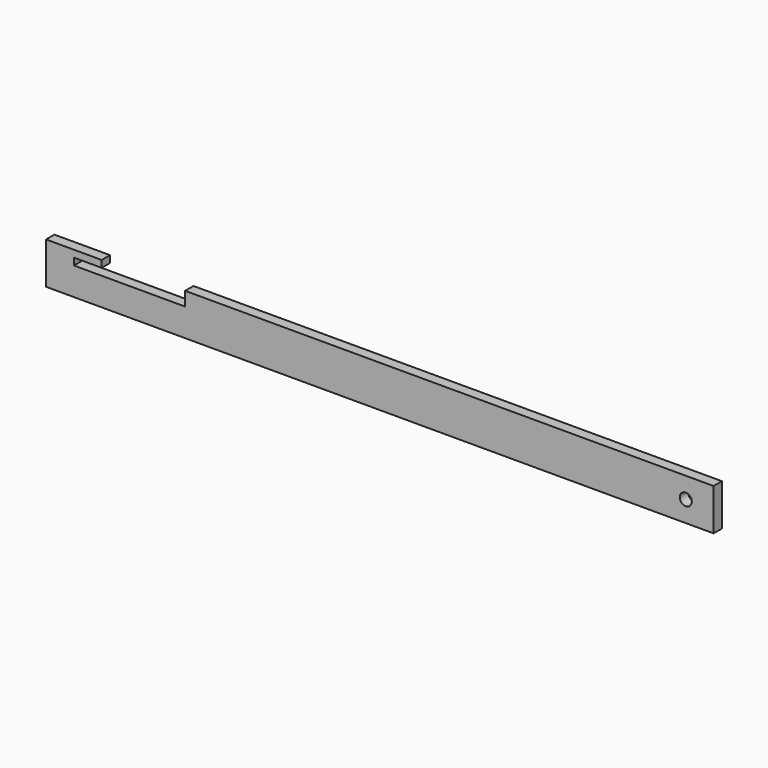
from build123d import *

# Parameters (mm, degrees)
F0_W     = 101.6
F0_H     = 44.45
F1_DEPTH = 6.35
F2_W     = 609.6
F2_H     = 38.1
F2_W_2   = 101.6
F2_H_2   = 6.35
F3_DEPTH = 9.525
F4_DEPTH = 9.525
F6_W     = 76.2
F6_H     = 25.4
F7_DEPTH = 25.4
F8_R     = 5.5
F9_DEPTH = 25.4


# Not quite as in the source:
# - ends of sketch curves that miss each other by under 0.0002 mm in the source are joined


with BuildPart() as f1:
    # F0 (on Top) → F1 (new body)
    with BuildSketch(Plane.XY):
        with Locations((-3.1162388623, -13.4853734154)):
            Rectangle(F0_W, F0_H)
    extrude(amount=F1_DEPTH)

    # F2 (on face) → F4 (cut)
    with BuildSketch(Plane.XZ.offset(35.7103734154)):
        with Locations((-3.1162388623, 3.175)):
            Rectangle(F2_W_2, F2_H_2)
    extrude(amount=-F4_DEPTH, mode=Mode.SUBTRACT)


with BuildPart() as f3:
    # F2 (on face) → F3 (new body)
    with BuildSketch(Plane.XZ.offset(35.7103734154)):
        with Locations((225.4837611377, -6.35)):
            Rectangle(F2_W, F2_H)
        with Locations((-3.1162388623, 3.175)):
            Rectangle(F2_W_2, F2_H_2, mode=Mode.SUBTRACT)
    extrude(amount=-F3_DEPTH)

    # F6 (on face) → F7 (cut)
    with BuildSketch(Plane.XZ.offset(35.7103734154)):
        with Locations((9.5837611377, 19.05)):
            Rectangle(F6_W, F6_H)
    extrude(amount=-F7_DEPTH, mode=Mode.SUBTRACT)

    # F8 (on face) → F9 (cut)
    with BuildSketch(Plane.XZ.offset(35.7103734154)):
        with Locations((504.8837611377, -6.35)):
            Circle(F8_R)
    extrude(amount=-F9_DEPTH, mode=Mode.SUBTRACT)


solid = f3.part
